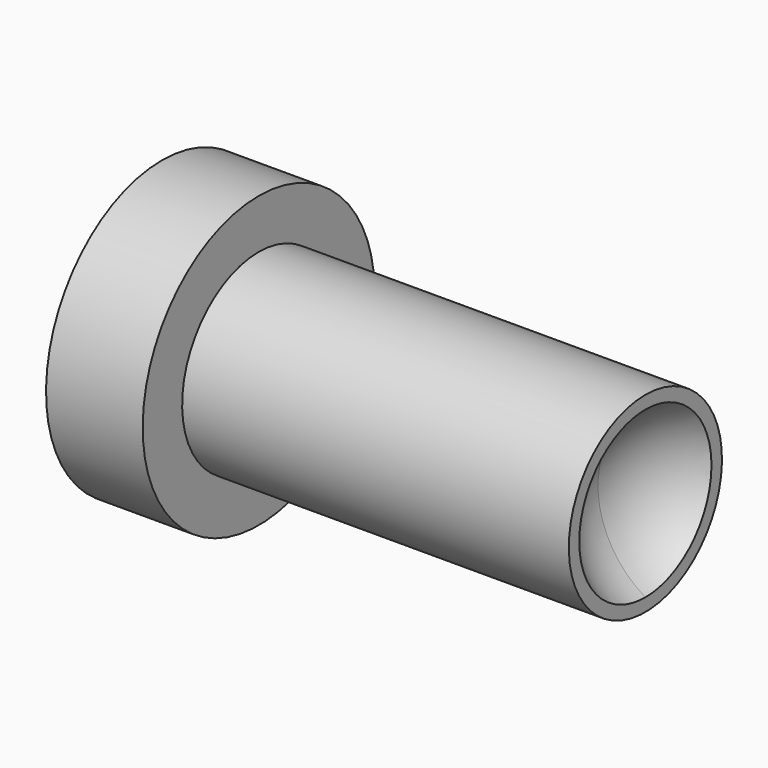
from build123d import *
from build123d import SkipClean  # not in build123d's __all__


with BuildPart() as f1:
    # F0 (on Front) → F1 (revolve)
    with BuildSketch(Plane.XZ):
        Polygon((63.5, 12.573), (12.7, 12.573), (12.7, 19.05), (0, 19.05), (0, 0), (63.5, 0), align=None)
    revolve(axis=Axis((25.1227524132, 0, 0), (1, 0, 0)))

    # F2 (on Front) → F3 (revolve, cut)
    with BuildSketch(Plane.XZ):
        with BuildLine():
            Line((69.85, -12.573), (69.85, 12.573))
            ThreePointArc((69.85, 12.573), (57.277, 0), (69.85, -12.573))
        make_face()
    with SkipClean():  # cleaning this boolean's faces spoils the solid; the shape is the same uncleaned
        revolve(axis=Axis((69.85, 0, 6.9150045632), (0, 0, -1)), mode=Mode.SUBTRACT)


solid = f1.part
